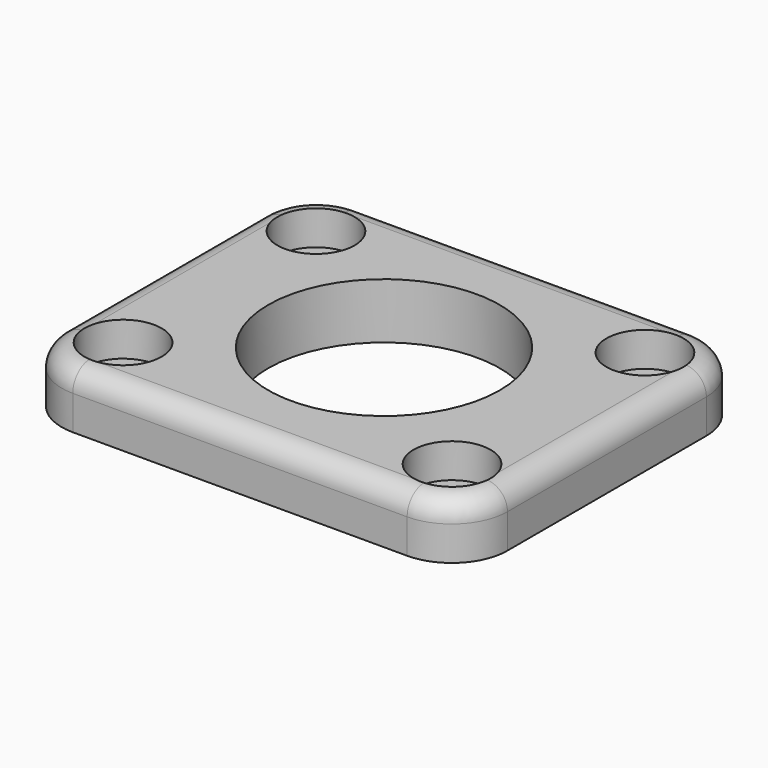
from build123d import *

# Parameters (mm, degrees)
F0_W          = 104
F0_H          = 84
F1_DEPTH      = 13
F3_R          = 9
F4_DEPTH      = 8
F5_R          = 4.5
F6_DEPTH      = 25
F7_R          = 27
F8_DEPTH      = 25
F9_R          = 13
F10_T1_DEPTH  = 58
F10_T3_DEPTH  = 78
F10_T6_ANGLE  = 90
F10_T8_ANGLE  = 90
F10_T10_ANGLE = 90
F10_T12_ANGLE = 90


# Not quite as in the source:
# - a fillet or chamfer that OpenCascade refuses, or shapes differently, is made with other operations: its cross-section is extruded or revolved along the edge and cut away or added


with BuildPart() as f1:
    # F0 (on Top) → F1 (new body)
    with BuildSketch(Plane.XY):
        Rectangle(F0_W, F0_H)
    extrude(amount=-F1_DEPTH)

    # F3 (on Top) → F4 (cut)
    with BuildSketch(Plane.XY):
        with Locations((38.3695703445, 28.125)):
            Circle(F3_R)
        with Locations((38.3695703445, -28.125)):
            Circle(F3_R)
        with Locations((-38.3695703445, 28.125)):
            Circle(F3_R)
        with Locations((-38.3695703445, -28.125)):
            Circle(F3_R)
    extrude(amount=-F4_DEPTH, mode=Mode.SUBTRACT)

    # F5 (on face) → F6 (cut)
    with BuildSketch(Plane.XY.offset(-8)):
        with Locations((38.3695703445, 28.125)):
            Circle(F5_R)
        with Locations((38.3695703445, -28.125)):
            Circle(F5_R)
        with Locations((-38.3695703445, 28.125)):
            Circle(F5_R)
        with Locations((-38.3695703445, -28.125)):
            Circle(F5_R)
    extrude(amount=-F6_DEPTH, mode=Mode.SUBTRACT)

    # F7 (on Top) → F8 (cut)
    with BuildSketch(Plane.XY):
        Circle(F7_R)
    extrude(amount=-F8_DEPTH, mode=Mode.SUBTRACT)

    # F9
    f9_edges = [f1.edges().sort_by_distance(p)[0] for p in [
        (-52, 42, -6.5),
        (-52, -42, -6.5),
        (52, -42, -6.5),
        (52, 42, -6.5),
    ]]
    fillet(f9_edges, radius=F9_R)

    # F10: fillet of radius 5 on 8 edges, made by hand

    # F10_s2 → F10_t1 (cut)
    with BuildSketch(Plane.XZ.offset(-29)):
        with BuildLine():
            ThreePointArc((-47, 0), (-50.5355339059, -1.4644660941), (-52, -5))
            Line((-52, -5), (-52, 0))
            Line((-52, 0), (-47, 0))
        make_face()
        with BuildLine():
            ThreePointArc((52, -5), (50.5355339059, -1.4644660941), (47, 0))
            Line((47, 0), (52, 0))
            Line((52, 0), (52, -5))
        make_face()
    extrude(amount=F10_T1_DEPTH, mode=Mode.SUBTRACT)

    # F10_s4 → F10_t3 (cut)
    with BuildSketch(Plane.YZ.offset(-39)):
        with BuildLine():
            ThreePointArc((-37, 0), (-40.5355339059, -1.4644660941), (-42, -5))
            Line((-42, -5), (-42, 0))
            Line((-42, 0), (-37, 0))
        make_face()
        with BuildLine():
            ThreePointArc((37, 0), (40.5355339059, -1.4644660941), (42, -5))
            Line((42, -5), (42, 0))
            Line((42, 0), (37, 0))
        make_face()
    extrude(amount=F10_T3_DEPTH, mode=Mode.SUBTRACT)

    # F10_s5 → F10_t6 (revolve, cut)
    with BuildSketch(Plane.XZ.offset(29)):
        with BuildLine():
            ThreePointArc((47, 0), (50.5355339059, -1.4644660941), (52, -5))
            Line((52, -5), (52, 0))
            Line((52, 0), (47, 0))
        make_face()
    revolve(axis=Axis((39, -29, 0), (0, 0, -1)), revolution_arc=F10_T6_ANGLE, mode=Mode.SUBTRACT)

    # F10_s7 → F10_t8 (revolve, cut)
    with BuildSketch(Plane.XZ.offset(-29)):
        with BuildLine():
            ThreePointArc((47, 0), (50.5355339059, -1.4644660941), (52, -5))
            Line((52, -5), (52, 0))
            Line((52, 0), (47, 0))
        make_face()
    revolve(axis=Axis((39, 29, 0), (0, 0, 1)), revolution_arc=F10_T8_ANGLE, mode=Mode.SUBTRACT)

    # F10_s9 → F10_t10 (revolve, cut)
    with BuildSketch(Plane.YZ.offset(-39)):
        with BuildLine():
            ThreePointArc((-37, 0), (-40.5355339059, -1.4644660941), (-42, -5))
            Line((-42, -5), (-42, 0))
            Line((-42, 0), (-37, 0))
        make_face()
    revolve(axis=Axis((-39, -29, 0), (0, 0, -1)), revolution_arc=F10_T10_ANGLE, mode=Mode.SUBTRACT)

    # F10_s11 → F10_t12 (revolve, cut)
    with BuildSketch(Plane.YZ.offset(-39)):
        with BuildLine():
            ThreePointArc((37, 0), (40.5355339059, -1.4644660941), (42, -5))
            Line((42, -5), (42, 0))
            Line((42, 0), (37, 0))
        make_face()
    revolve(axis=Axis((-39, 29, 0), (0, 0, 1)), revolution_arc=F10_T12_ANGLE, mode=Mode.SUBTRACT)


solid = f1.part
